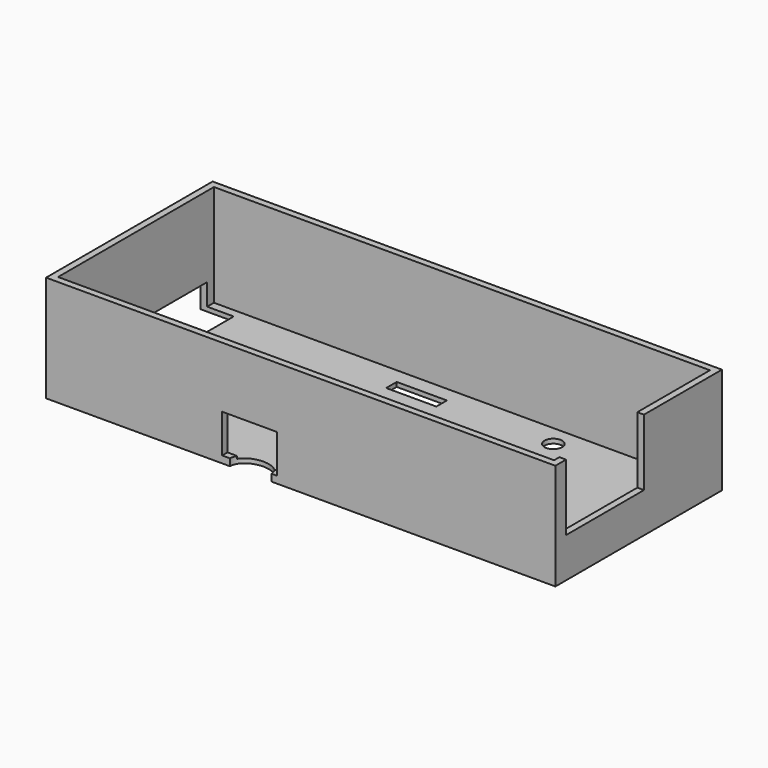
from build123d import *

# Parameters (mm, degrees)
F0_W      = 115
F0_H      = 47
F0_W_2    = 112
F0_H_2    = 44
F1_DEPTH  = 1
F2_W      = 115
F2_H      = 47
F2_W_2    = 112
F2_H_2    = 44
F3_DEPTH  = 8
F5_DEPTH  = 15
F6_R      = 2
F6_W      = 11.0119888559
F6_H      = 3.023254365
F6_W_2    = 11.3270477741
F6_H_2    = 2.977441065
F7_DEPTH  = 5
F8_W      = 12.3954089358
F8_H      = 8.6996963946
F9_DEPTH  = 5
F11_W     = 18.856737297
F11_H     = 5.874496419
F12_DEPTH = 7.5
F13_W     = 21.3697072027
F13_H     = 2
F14_DEPTH = 5
F15_DEPTH = 4


# Not quite as in the source:
# - a feature names something its author has since deleted; it is built from what else it names


with BuildPart() as f1:
    # F0 (on Top) → F1 (new body)
    with BuildSketch(Plane.XY):
        Rectangle(F0_W, F0_H)
        Rectangle(F0_W_2, F0_H_2, mode=Mode.SUBTRACT)
        Rectangle(F0_W_2, F0_H_2)
    extrude(amount=F1_DEPTH)

    # F2 (on face) → F3 (join)
    with BuildSketch(Plane.XY.offset(1)):
        Rectangle(F2_W, F2_H)
        Rectangle(F2_W_2, F2_H_2, mode=Mode.SUBTRACT)
    extrude(amount=F3_DEPTH)

    # F4 (on face) → F5 (join)
    with BuildSketch(Plane.XY.offset(9)):
        Polygon((57.5, -20.5), (56, -20.5), (56, -22), (-56, -22), (-56, 22), (56, 22), (56, 1.5), (57.5, 1.5), (57.5, 23.5), (-57.5, 23.5), (-57.5, -23.5), (57.5, -23.5), align=None)
    extrude(amount=F5_DEPTH)

    # F6 (on face) → F7 (cut)
    with BuildSketch(Plane(origin=(0, 0, 0), x_dir=(1, 0, 0), z_dir=(0, 0, -1))):
        with Locations((24.4, -17.3)):
            Circle(F6_R)
        with Locations((21.9000000507, -5.4)):
            Circle(F6_R)
        with Locations((22.334024366, -0.8409991293)):
            Rectangle(F6_W, F6_H)
        with Locations((-6.2833959528, -17.0318004675)):
            Rectangle(F6_W_2, F6_H_2)
    extrude(amount=-F7_DEPTH, mode=Mode.SUBTRACT)

    # F8 (on face) → F9 (cut)
    with BuildSketch(Plane.XZ.offset(23.5)):
        with Locations((-11.533238925, 5.9268509503)):
            Rectangle(F8_W, F8_H)
    extrude(amount=-F9_DEPTH, mode=Mode.SUBTRACT)

    # F11 (on face) → F12 (cut)
    with BuildSketch(Plane(origin=(-57.5, 0, 0), x_dir=(0, -1, 0), z_dir=(-1, 0, 0))):
        with Locations((-10.6531684287, 2.9372482095)):
            Rectangle(F11_W, F11_H)
    extrude(amount=-F12_DEPTH, mode=Mode.SUBTRACT)

    # F13 (on face) → F14 (cut)
    with BuildSketch(Plane.YZ.offset(57.5)):
        with Locations((-9.4148694571, 10)):
            Rectangle(F13_W, F13_H)
    extrude(amount=-F14_DEPTH, mode=Mode.SUBTRACT)

    # F10 (on face) → F15 (cut)
    with BuildSketch(Plane(origin=(0, 0, 0), x_dir=(1, 0, 0), z_dir=(0, 0, -1))):
        with BuildLine():
            add(Edge.make_bspline(
                [(-15.979938673, 23.5), (-15.979938673, 19.9097213669), (-11.31611038, 19.9097213669), (-6.652282087, 19.9097213669), (-6.652282087, 23.5)],
                knots=[3.1415926536, 3.1415926536, 3.1415926536, 4.7123889804, 4.7123889804, 6.2831853072, 6.2831853072, 6.2831853072], degree=2, weights=[1, 0.7071067812, 1, 0.7071067812, 1]))
            Line((-6.652282087, 23.5), (-15.979938673, 23.5))
        make_face()
    extrude(amount=-F15_DEPTH, mode=Mode.SUBTRACT)


solid = f1.part
